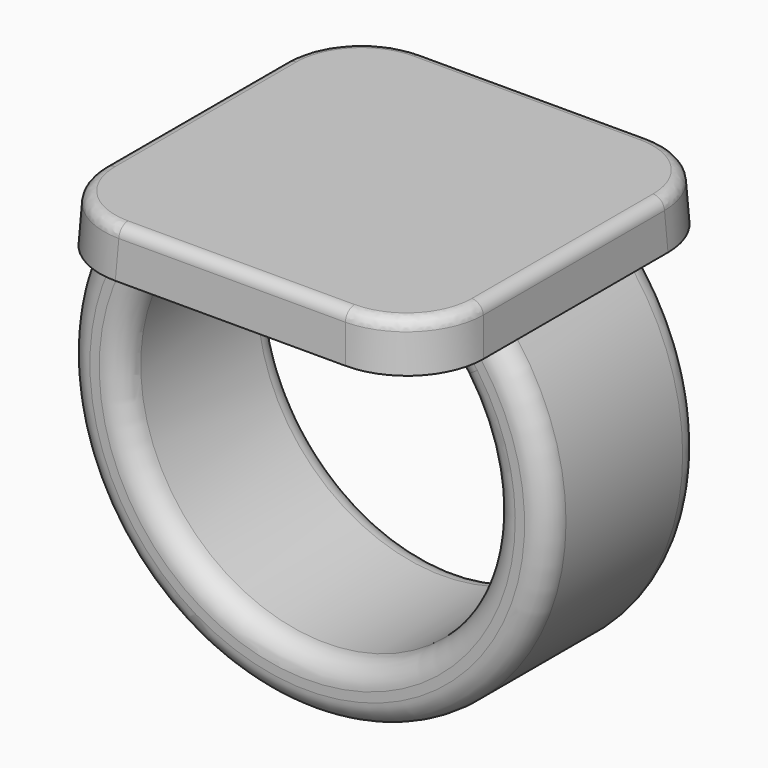
from build123d import *

# Parameters (mm, degrees)
F0_W          = 25.4
F0_H          = 25.4
F1_DEPTH      = 3.175
F1_TAPER      = 3
F3_W          = 5.08
F3_H          = 12.7
F6_DEPTH      = 6.35
F6_DEPTH_BACK = 6.35
F7_R          = 5.08
F8_R          = 1.524
F9_R          = 0.762


with BuildPart() as f1:
    # F0 (on Top) → F1 (new body)
    with BuildSketch(Plane.XY):
        Rectangle(F0_W, F0_H)
    extrude(amount=F1_DEPTH, taper=F1_TAPER)

    # F4: sweep along a path in F2
    with BuildLine(Plane.XZ) as f4_path:
        ThreePointArc((-10.16, 0), (0, -23.5582897328), (10.16, 0))
    # F3 (on face) → F4 (sweep)
    with BuildSketch(Plane(origin=(0, 0, 0), x_dir=(1, 0, 0), z_dir=(0, 0, -1))):
        with Locations((-10.16, 0)):
            Rectangle(F3_W, F3_H)
    sweep(path=f4_path.line)

    # F5 (on Front) → F6 (join, two sides)
    with BuildSketch(Plane.XZ) as f6_sk:
        with BuildLine():
            Line((10.0130578512, -2.535746045), (10.16, 0))
            Line((10.16, 0), (7.62, 0))
            ThreePointArc((7.62, 0), (8.9072265211, -1.1822790439), (10.0130578512, -2.535746045))
        make_face()
    extrude(amount=F6_DEPTH)
    extrude(f6_sk.sketch, amount=-F6_DEPTH_BACK)

    # F7
    f7_edges = [f1.edges().sort_by_distance(p)[0] for p in [
        (12.616803, -12.616803, 1.5875),
        (12.616803, 12.616803, 1.5875),
        (-12.616803, 12.616803, 1.5875),
        (-12.616803, -12.616803, 1.5875),
    ]]
    fillet(f7_edges, radius=F7_R)

    # F8
    f8_edges = [f1.edges().sort_by_distance(p)[0] for p in [
        (-1.743325, -6.35, -21.711017),
        (8.907227, -6.35, -1.182279),
        (-1.743325, 6.35, -21.711017),
        (0, -6.35, -25.501344),
        (0, 6.35, -25.501344),
        (8.907227, 6.35, -1.182279),
    ]]
    fillet(f8_edges, radius=F8_R)

    # F9
    f9_edges = [f1.edges().sort_by_distance(p)[0] for p in [
        (12.533605, 0, 3.175),
        (11.048589, -11.048589, 3.175),
        (11.048589, 11.048589, 3.175),
        (0, -12.533605, 3.175),
        (0, 12.533605, 3.175),
        (-11.048589, -11.048589, 3.175),
        (-11.048589, 11.048589, 3.175),
        (-12.533605, 0, 3.175),
    ]]
    fillet(f9_edges, radius=F9_R)


solid = f1.part
